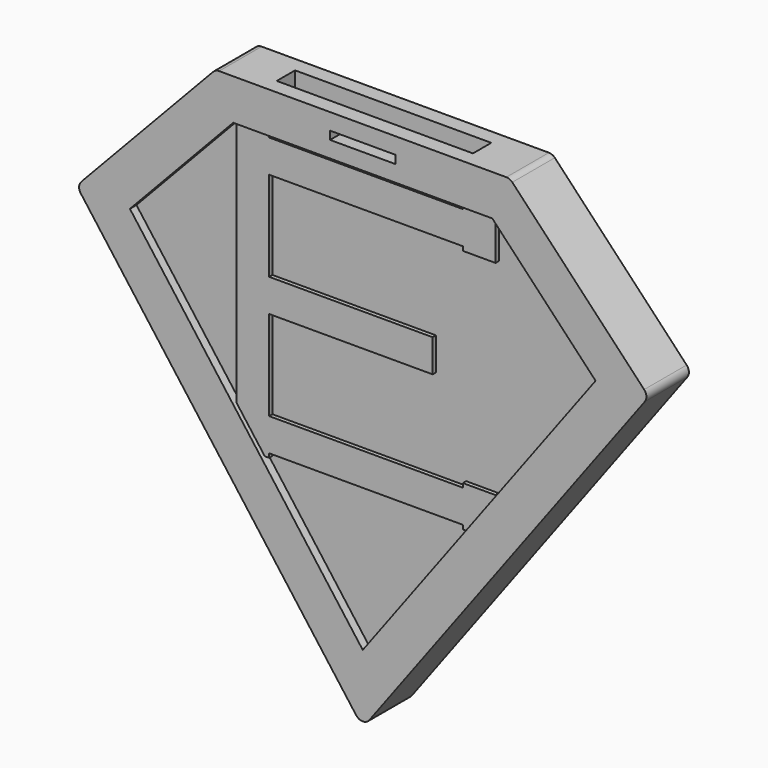
from build123d import *

# Parameters (mm, degrees)
F1_DEPTH  = 3.25
F3_DEPTH  = 0.5
F5_DEPTH  = 0.5
F6_W      = 23.6895351076
F6_H      = 0.5
F7_DEPTH  = 0.5
F8_W      = 23.6895351076
F8_H      = 0.5000002682
F9_DEPTH  = 0.5
F10_W     = 24
F10_H     = 2.8
F11_DEPTH = 20
F13_DEPTH = 1.4
F14_W     = 8
F14_H     = 1
F15_DEPTH = 25
F16_R     = 1


# Not quite as in the source:
# - ends of sketch curves that miss each other by under 0.0002 mm in the source are joined


with BuildPart() as f1:
    # F0 (on Front) → F1 (new body, symmetric)
    with BuildSketch(Plane.XZ):
        Polygon((18, 18), (0, 18), (-18, 18), (-35, 0), (0, -47), (35, 0), align=None)
    extrude(amount=F1_DEPTH, both=True)

    # F2 (on face) → F3 (cut)
    with BuildSketch(Plane.XZ.offset(3.25)):
        Polygon((15.8447675538, 13), (-15.8447675538, 13), (-28.4822773709, -0.3808927475), (1.162e-07, -38.628522516), (28.4822775009, -0.3808928851), align=None)
    extrude(amount=-F3_DEPTH, mode=Mode.SUBTRACT)

    # F4 (on face) → F5 (cut)
    with BuildSketch(Plane(origin=(0, 3.25, 0), x_dir=(-1, 0, 0), z_dir=(0, 1, 0))):
        Polygon((28.482277527, -0.3808925379), (15.8447676545, 13.0000002682), (-15.8447670441, 13.0000002682), (-28.4822772579, -0.3808928993), (0, -38.6285223599), align=None)
    extrude(amount=-F5_DEPTH, mode=Mode.SUBTRACT)

    # F6 (on face) → F7 (cut)
    with BuildSketch(Plane.XZ.offset(2.75)):
        Polygon((-15.8447675538, -17.3512630734), (-15.8447675538, 13), (-28.4822773709, -0.3808927475), align=None)
        Polygon((28.4822775009, -0.3808928851), (15.8447675538, 13), (15.8447675538, 8), (11.8447675538, 8), (11.8447675538, 8.5), (-11.8447675538, 8.5), (-11.8447675538, -2.5), (8.1552324462, -2.5), (8.1552324462, -6.5), (-11.8447675538, -6.5), (-11.8447675538, -17.5), (11.8447675538, -17.5), (11.8447675538, -17), (15.8447675538, -17), (15.8447675538, -17.3512633855), align=None)
        with Locations((0, 12.75)):
            Rectangle(F6_W, F6_H)
        Polygon((-11.8447675538, -22), (-12.3829421829, -22), (1.162e-07, -38.628522516), (12.3829424153, -22), (11.8447675538, -22), (11.8447675538, -21.5), (-11.8447675538, -21.5), align=None)
    extrude(amount=-F7_DEPTH, mode=Mode.SUBTRACT)

    # F8 (on face) → F9 (cut)
    with BuildSketch(Plane(origin=(0, 2.75, 0), x_dir=(-1, 0, 0), z_dir=(0, 1, 0))):
        Polygon((-11.8447675538, -2.5), (8.1552324462, -2.5), (8.1552324462, -6.5), (-11.8447675538, -6.5), (-11.8447675538, -17.5), (11.8447675538, -17.5), (11.8447675538, -17), (15.8447675538, -17), (15.8447675538, -17.3512630734), (28.482277527, -0.3808925379), (15.8447676545, 13.0000002682), (15.8447675538, 8), (11.8447675538, 8), (11.8447675538, 8.5), (-11.8447675538, 8.5), align=None)
        Polygon((11.8447675538, -21.5), (-11.8447675538, -21.5), (-11.8447675538, -22), (-12.3829424153, -22), (0, -38.6285223599), (12.3829421829, -22), (11.8447675538, -22), align=None)
        Polygon((-15.8447675538, -17.3512630734), (-15.8447675538, 13), (-28.4822772579, -0.3808928993), align=None)
        with Locations((0, 12.7500001341)):
            Rectangle(F8_W, F8_H)
    extrude(amount=-F9_DEPTH, mode=Mode.SUBTRACT)

    # F10 (on face) → F11 (cut)
    with BuildSketch(Plane.XY.offset(18)):
        Rectangle(F10_W, F10_H)
    extrude(amount=-F11_DEPTH, mode=Mode.SUBTRACT)

    # F12 (on Front) → F13 (cut, symmetric)
    with BuildSketch(Plane.XZ):
        with BuildLine():
            Line((12, -2), (-12, -2))
            ThreePointArc((-12, -2), (0, -14), (12, -2))
        make_face()
    extrude(amount=F13_DEPTH, both=True, mode=Mode.SUBTRACT)

    # F14 (on face) → F15 (cut)
    with BuildSketch(Plane.XZ.offset(3.25)):
        with Locations((0, 15.5)):
            Rectangle(F14_W, F14_H)
    extrude(amount=-F15_DEPTH, mode=Mode.SUBTRACT)

    # F16
    f16_edges = [f1.edges().sort_by_distance(p)[0] for p in [
        (0, 0, -47),
        (35, 0, 0),
        (-35, 0, 0),
        (-18, 0, 18),
        (18, 0, 18),
    ]]
    fillet(f16_edges, radius=F16_R)


solid = f1.part
